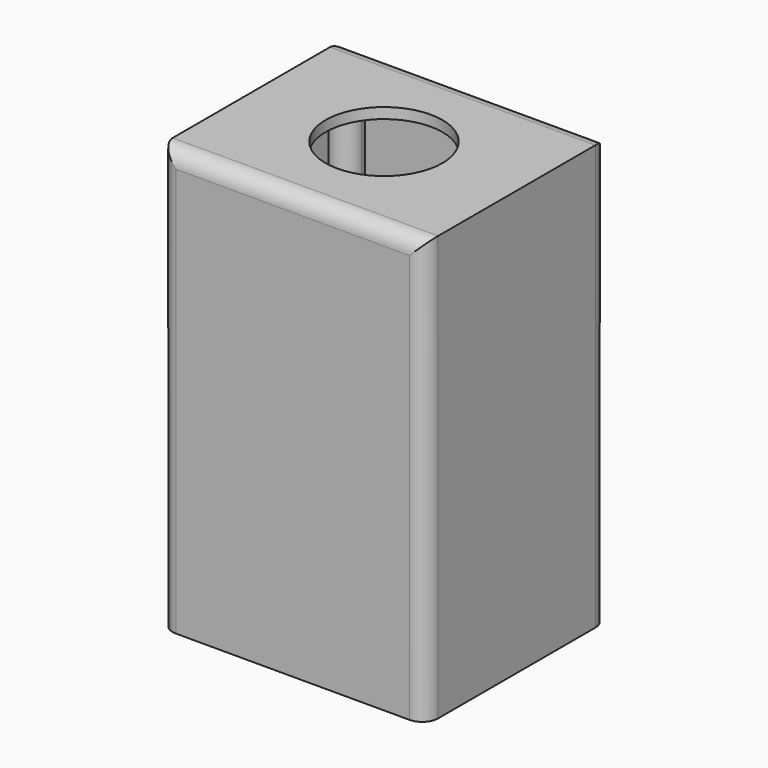
from build123d import *

# Parameters (mm, degrees)
F0_W     = 50
F0_H     = 43
F0_R     = 1.5
F1_DEPTH = 80
F3_T     = -2
F2_R     = 11
F4_DEPTH = 3.1
F5_R     = 3
F6_R     = 1.5
F7_DEPTH = 77
F8_DEPTH = 40


# Not quite as in the source:
# - a feature names something its author has since deleted; it is built from what else it names


with BuildPart() as f1:
    # F0 (on Top) → F1 (new body)
    with BuildSketch(Plane.XY):
        with Locations((-9.0278687937, 4.7237686813)):
            Rectangle(F0_W, F0_H)
        with Locations((-31.0278687937, -13.7762313187)):
            Circle(F0_R, mode=Mode.SUBTRACT)
        with Locations((12.9721312063, -13.7762313187)):
            Circle(F0_R, mode=Mode.SUBTRACT)
        with Locations((-31.0278687937, 23.2237686813)):
            Circle(F0_R, mode=Mode.SUBTRACT)
        with Locations((12.9721312063, 23.2237686813)):
            Circle(F0_R, mode=Mode.SUBTRACT)
        with Locations((12.9721312063, 23.2237686813)):
            Circle(F0_R)
        with Locations((12.9721312063, -13.7762313187)):
            Circle(F0_R)
        with Locations((-31.0278687937, -13.7762313187)):
            Circle(F0_R)
        with Locations((-31.0278687937, 23.2237686813)):
            Circle(F0_R)
    extrude(amount=F1_DEPTH)

    # F3
    f3_openings = [f1.faces().sort_by_distance(p)[0] for p in [
        (-9.027869, 4.723769, 0),
    ]]
    offset(amount=F3_T, openings=f3_openings)

    # F2 (on face) → F4 (cut)
    with BuildSketch(Plane.XY.offset(80)):
        with Locations((-9.0278687937, 4.7237686813)):
            Circle(F2_R)
    extrude(amount=-F4_DEPTH, mode=Mode.SUBTRACT)

    # F5
    f5_edges = [f1.edges().sort_by_distance(p)[0] for p in [
        (15.972131, 26.223769, 40),
        (-9.027869, 26.223769, 80),
        (-34.027869, 26.223769, 40),
        (15.972131, -16.776231, 40),
        (-9.027869, -16.776231, 80),
        (-34.027869, -16.776231, 40),
    ]]
    fillet(f5_edges, radius=F5_R)

    # F6 (on face) → F7 (join)
    with BuildSketch(Plane.XY):
        with BuildLine():
            ThreePointArc((12.9721312104, -16.7762313187), (15.0934515513, -15.8975516608), (15.9721312063, -13.7762313187))
            ThreePointArc((15.9721312063, -13.7762313187), (10.8508108613, -11.6549109766), (12.9721312104, -16.7762313187))
        make_face()
        with Locations((12.9721312063, -13.7762313187)):
            Circle(F6_R, mode=Mode.SUBTRACT)
        with BuildLine():
            ThreePointArc((12.9721312063, 26.2237686813), (10.8508108627, 21.1024483377), (15.9721312063, 23.2237686813))
            ThreePointArc((15.9721312063, 23.2237686813), (15.0934515498, 25.3450890248), (12.9721312063, 26.2237686813))
        make_face()
        with Locations((12.9721312063, 23.2237686813)):
            Circle(F6_R, mode=Mode.SUBTRACT)
        with BuildLine():
            ThreePointArc((-34.0278687937, -13.776231286), (-33.1491891488, -15.8975516507), (-31.0278687937, -16.7762313187))
            ThreePointArc((-31.0278687937, -16.7762313187), (-28.9065484502, -15.8975516623), (-28.0278687937, -13.7762313187))
            ThreePointArc((-28.0278687937, -13.7762313187), (-31.0278687774, -10.7762313187), (-34.0278687937, -13.776231286))
        make_face()
        with Locations((-31.0278687937, -13.7762313187)):
            Circle(F6_R, mode=Mode.SUBTRACT)
        with BuildLine():
            ThreePointArc((-28.0278687937, 23.2237686813), (-28.9065484366, 25.3450890113), (-31.0278687555, 26.2237686813))
            ThreePointArc((-31.0278687555, 26.2237686813), (-33.1491891237, 25.3450890384), (-34.0278687937, 23.2237686813))
            ThreePointArc((-34.0278687937, 23.2237686813), (-31.0278687937, 20.2237686813), (-28.0278687937, 23.2237686813))
        make_face()
        with Locations((-31.0278687937, 23.2237686813)):
            Circle(F6_R, mode=Mode.SUBTRACT)
    extrude(amount=F7_DEPTH)

    # F0 (on Top) → F8 (cut)
    with BuildSketch(Plane.XY):
        with Locations((-31.0278687937, 23.2237686813)):
            Circle(F0_R)
        with Locations((12.9721312063, 23.2237686813)):
            Circle(F0_R)
        with Locations((-31.0278687937, -13.7762313187)):
            Circle(F0_R)
        with Locations((12.9721312063, -13.7762313187)):
            Circle(F0_R)
    extrude(amount=F8_DEPTH, mode=Mode.SUBTRACT)


solid = f1.part
